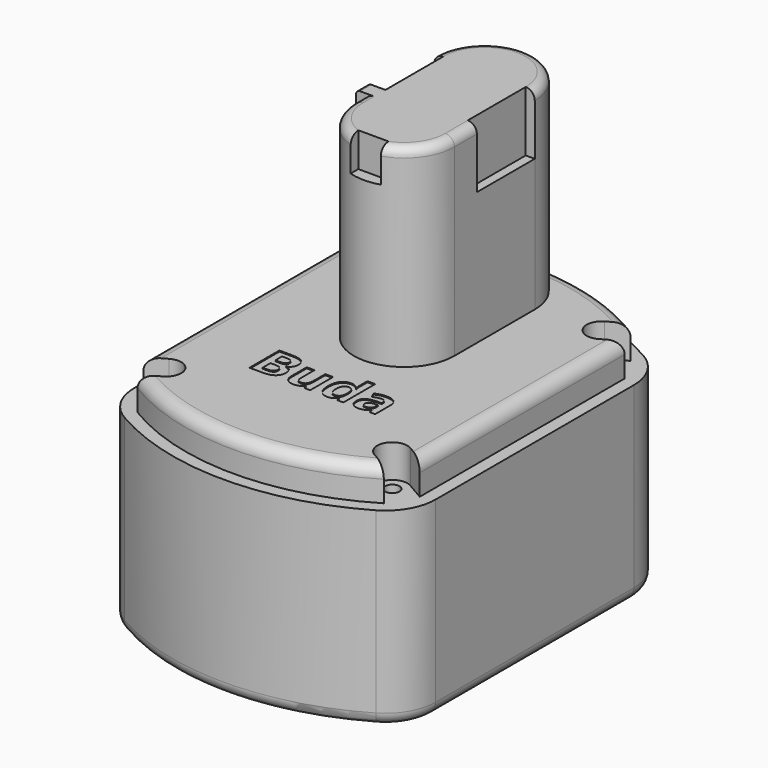
from build123d import *

# Parameters (mm, degrees)
F1_DEPTH      = 48.26
F3_DEPTH      = 8.382
F5_DEPTH      = 8.382
F6_R          = 1.8288
F7_DEPTH      = 32.8422
F9_DEPTH      = 57.15
F10_W         = 2.286
F10_H         = 3.556
F11_DEPTH     = 48.768
F12_R         = 2.286
F13_W         = 2.286
F13_H         = 18.288
F14_DEPTH     = 15.24
F16_DEPTH     = 8.636
F17_R         = 1.016
F18_TEXT_SIZE = 13.2291666667
F19_DEPTH     = 0.254
F20_R         = 12.7
F21_R         = 3.048
F22_R         = 3.175


# Not quite as in the source:
# - Text() gives the source's letters only with a copy of the font that has no kerning and outlines rounded to 1/6400 em; it was checked with that copy


with BuildPart() as f1:
    # F0 (on Top) → F1 (new body)
    with BuildSketch(Plane.XY):
        with BuildLine():
            Line((38.1, -38.1), (38.1, 38.1))
            ThreePointArc((38.1, 38.1), (0, 50.8), (-38.1, 38.1))
            Line((-38.1, 38.1), (-38.1, -38.1))
            ThreePointArc((-38.1, -38.1), (0, -50.8), (38.1, -38.1))
        make_face()
    extrude(amount=-F1_DEPTH)

    # F2 (on face) → F3 (join)
    with BuildSketch(Plane.XY):
        with BuildLine():
            Line((34.925, -36.4868884968), (34.925, 36.4868884968))
            ThreePointArc((34.925, 36.4868884968), (0, 47.625), (-34.925, 36.4868884968))
            Line((-34.925, 36.4868884968), (-34.925, -36.4868884968))
            ThreePointArc((-34.925, -36.4868884968), (0, -47.625), (34.925, -36.4868884968))
        make_face()
    extrude(amount=F3_DEPTH)

    # F4 (on face) → F5 (cut, through all)
    with BuildSketch(Plane.XY.offset(8.382)):
        with BuildLine():
            ThreePointArc((-26.67, -36.3957567884), (-25.2754432116, -31.1912), (-30.48, -29.7966432116))
            Line((-30.48, -29.7966432116), (-52.4770452561, -42.4966432116))
            ThreePointArc((-52.4770452561, -42.4966432116), (-53.8716020445, -47.7012), (-48.6670452561, -49.0957567884))
            Line((-48.6670452561, -49.0957567884), (-26.67, -36.3957567884))
        make_face()
        with BuildLine():
            Line((52.4770452561, -42.4966432116), (30.48, -29.7966432116))
            ThreePointArc((30.48, -29.7966432116), (25.2754432116, -31.1912), (26.67, -36.3957567884))
            Line((26.67, -36.3957567884), (48.6670452561, -49.0957567884))
            ThreePointArc((48.6670452561, -49.0957567884), (53.8716020445, -47.7012), (52.4770452561, -42.4966432116))
        make_face()
        with BuildLine():
            Line((-52.4770452561, 42.4966432116), (-30.48, 29.7966432116))
            ThreePointArc((-30.48, 29.7966432116), (-25.2754432116, 31.1912), (-26.67, 36.3957567884))
            Line((-26.67, 36.3957567884), (-48.6670452561, 49.0957567884))
            ThreePointArc((-48.6670452561, 49.0957567884), (-53.8716020445, 47.7012), (-52.4770452561, 42.4966432116))
        make_face()
        with BuildLine():
            ThreePointArc((26.67, 36.3957567884), (25.2754432116, 31.1912), (30.48, 29.7966432116))
            Line((30.48, 29.7966432116), (52.4770452561, 42.4966432116))
            ThreePointArc((52.4770452561, 42.4966432116), (53.8716020445, 47.7012), (48.6670452561, 49.0957567884))
            Line((48.6670452561, 49.0957567884), (26.67, 36.3957567884))
        make_face()
    extrude(amount=-F5_DEPTH, mode=Mode.SUBTRACT)

    # F6 (on face) → F7 (cut)
    with BuildSketch(Plane.XY):
        with Locations((28.575, -33.0962)):
            Circle(F6_R)
        with Locations((28.575, 33.0962)):
            Circle(F6_R)
        with Locations((-28.575, 33.0962)):
            Circle(F6_R)
        with Locations((-28.575, -33.0962)):
            Circle(F6_R)
    extrude(amount=-F7_DEPTH, mode=Mode.SUBTRACT)

    # F8 (on Top) → F9 (join)
    with BuildSketch(Plane.XY):
        with BuildLine():
            ThreePointArc((-12.7, 6.35), (0, -6.35), (12.7, 6.35))
            Line((12.7, 6.35), (12.7, 31.75))
            ThreePointArc((12.7, 31.75), (0, 44.45), (-12.7, 31.75))
            Line((-12.7, 31.75), (-12.7, 6.35))
        make_face()
    extrude(amount=F9_DEPTH)

    # F10 (on face) → F11 (join, through all)
    with BuildSketch(Plane.XY.offset(8.382)):
        with Locations((-13.843, 11.684)):
            Rectangle(F10_W, F10_H)
    extrude(amount=F11_DEPTH)

    # F12
    f12_edges = [f1.edges().sort_by_distance(p)[0] for p in [
        (12.7, 19.05, 57.15),
    ]]
    fillet(f12_edges, radius=F12_R)

    # F13 (on face) → F14 (cut)
    with BuildSketch(Plane.XY.offset(57.15)):
        with Locations((11.557, 22.606)):
            Rectangle(F13_W, F13_H)
        with Locations((-11.557, 22.606)):
            Rectangle(F13_W, F13_H)
    extrude(amount=-F14_DEPTH, mode=Mode.SUBTRACT)

    # F15 (on face) → F16 (cut)
    with BuildSketch(Plane.XY.offset(57.15)):
        with BuildLine():
            Line((-3.81, -3.3420222864), (-3.81, -5.765027858))
            ThreePointArc((-3.81, -5.765027858), (0, -6.35), (3.81, -5.765027858))
            Line((3.81, -5.765027858), (3.81, -3.3420222864))
            Line((3.81, -3.3420222864), (-3.81, -3.3420222864))
        make_face()
    extrude(amount=-F16_DEPTH, mode=Mode.SUBTRACT)

    # F17
    f17_edges = [f1.edges().sort_by_distance(p)[0] for p in [
        (-14.986, 11.684, 57.15),
    ]]
    fillet(f17_edges, radius=F17_R)

    # F18 (on face) → F19 (cut)
    with BuildSketch(Plane.XY.offset(8.382)):
        with Locations((-16.9033610026, -22.86)):
            Text('Buda', F18_TEXT_SIZE, font='Open Sans', font_style=FontStyle.BOLD, text_align=(TextAlign.LEFT, TextAlign.BOTTOM))
    extrude(amount=-F19_DEPTH, mode=Mode.SUBTRACT)

    # F20
    f20_edges = [f1.edges().sort_by_distance(p)[0] for p in [
        (38.1, -38.1, -24.13),
        (38.1, 38.1, -24.13),
        (-38.1, -38.1, -24.13),
        (-38.1, 38.1, -24.13),
    ]]
    fillet(f20_edges, radius=F20_R)

    # F21
    f21_edges = [f1.edges().sort_by_distance(p)[0] for p in [
        (0, -47.625, 8.382),
        (34.925, 0, 8.382),
        (-34.925, 0, 8.382),
        (0, 47.625, 8.382),
    ]]
    fillet(f21_edges, radius=F21_R)

    # F22
    f22_edges = [f1.edges().sort_by_distance(p)[0] for p in [
        (38.1, 0, -48.26),
    ]]
    fillet(f22_edges, radius=F22_R)


solid = f1.part
